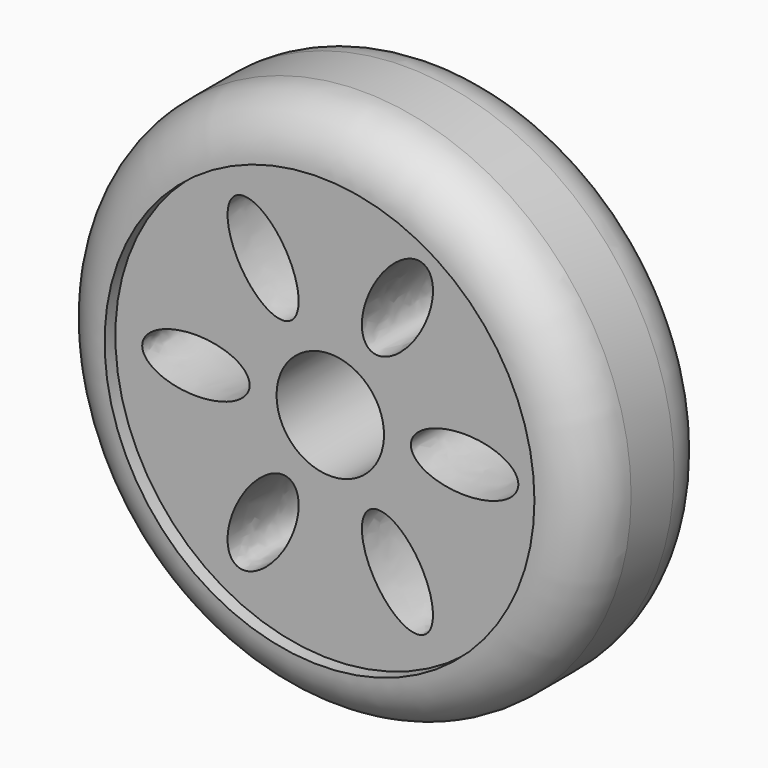
from build123d import *

# Parameters (mm, degrees)
F0_R     = 50
F0_R_2   = 40
F1_DEPTH = 15
F2_DEPTH = 12.5
F4_DEPTH = 25
F5_R     = 10
F6_DEPTH = 25
F7_R     = 9.99999


# Not quite as in the source:
# - a fillet or chamfer is up to 0.001 mm smaller than in the source, because OpenCascade refuses the exact size


with BuildPart() as f1:
    # F0 (on Front) → F1 (new body, symmetric)
    with BuildSketch(Plane.XZ):
        Circle(F0_R)
        Circle(F0_R_2, mode=Mode.SUBTRACT)
    extrude(amount=F1_DEPTH, both=True)

    # F0 (on Front) → F2 (join, symmetric)
    with BuildSketch(Plane.XZ):
        Circle(F0_R_2)
    extrude(amount=F2_DEPTH, both=True)

    # F3 (on face) → F4 (cut, through all)
    with BuildSketch(Plane(origin=(0, 12.5, 0), x_dir=(-1, 0, 0), z_dir=(0, 1, 0))):
        with BuildLine():
            add(Edge.make_bspline(
                [(7.5, 12.9903810568), (15, 8.6602540378), (18.75, 23.8156986041), (22.5, 38.9711431703), (11.25, 28.145825623), (0, 17.3205080757), (7.5, 12.9903810568)],
                knots=[0, 0, 0, 2.0943951024, 2.0943951024, 4.1887902048, 4.1887902048, 6.2831853072, 6.2831853072, 6.2831853072], degree=2, weights=[1, 0.5, 1, 0.5, 1, 0.5, 1]))
        make_face()
        with BuildLine():
            add(Edge.make_bspline(
                [(15, 0), (15, -8.6602540378), (30, -4.3301270189), (45, 0), (30, 4.3301270189), (15, 8.6602540378), (15, 0)],
                knots=[0, 0, 0, 2.0943951024, 2.0943951024, 4.1887902048, 4.1887902048, 6.2831853072, 6.2831853072, 6.2831853072], degree=2, weights=[1, 0.5, 1, 0.5, 1, 0.5, 1]))
        make_face()
        with BuildLine():
            add(Edge.make_bspline(
                [(7.5, -12.9903810568), (0, -17.3205080757), (11.25, -28.145825623), (22.5, -38.9711431703), (18.75, -23.8156986041), (15, -8.6602540378), (7.5, -12.9903810568)],
                knots=[0, 0, 0, 2.0943951024, 2.0943951024, 4.1887902048, 4.1887902048, 6.2831853072, 6.2831853072, 6.2831853072], degree=2, weights=[1, 0.5, 1, 0.5, 1, 0.5, 1]))
        make_face()
        with BuildLine():
            add(Edge.make_bspline(
                [(-7.5, -12.9903810568), (-15, -8.6602540378), (-18.75, -23.8156986041), (-22.5, -38.9711431703), (-11.25, -28.145825623), (0, -17.3205080757), (-7.5, -12.9903810568)],
                knots=[0, 0, 0, 2.0943951024, 2.0943951024, 4.1887902048, 4.1887902048, 6.2831853072, 6.2831853072, 6.2831853072], degree=2, weights=[1, 0.5, 1, 0.5, 1, 0.5, 1]))
        make_face()
        with BuildLine():
            add(Edge.make_bspline(
                [(-15, 0), (-15, 8.6602540378), (-30, 4.3301270189), (-45, 0), (-30, -4.3301270189), (-15, -8.6602540378), (-15, 0)],
                knots=[0, 0, 0, 2.0943951024, 2.0943951024, 4.1887902048, 4.1887902048, 6.2831853072, 6.2831853072, 6.2831853072], degree=2, weights=[1, 0.5, 1, 0.5, 1, 0.5, 1]))
        make_face()
        with BuildLine():
            add(Edge.make_bspline(
                [(-7.5, 12.9903810568), (0, 17.3205080757), (-11.25, 28.145825623), (-22.5, 38.9711431703), (-18.75, 23.8156986041), (-15, 8.6602540378), (-7.5, 12.9903810568)],
                knots=[0, 0, 0, 2.0943951024, 2.0943951024, 4.1887902048, 4.1887902048, 6.2831853072, 6.2831853072, 6.2831853072], degree=2, weights=[1, 0.5, 1, 0.5, 1, 0.5, 1]))
        make_face()
    extrude(amount=-F4_DEPTH, mode=Mode.SUBTRACT)

    # F5 (on face) → F6 (cut, through all)
    with BuildSketch(Plane(origin=(0, 12.5, 0), x_dir=(-1, 0, 0), z_dir=(0, 1, 0))):
        Circle(F5_R)
    extrude(amount=-F6_DEPTH, mode=Mode.SUBTRACT)

    # F7 (radius 10 in the source; OpenCascade refuses exactly that, so slightly less here)
    f7_edges = [f1.edges().sort_by_distance(p)[0] for p in [
        (-50, 15, 0),
        (-50, -15, 0),
    ]]
    fillet(f7_edges, radius=F7_R)


solid = f1.part
